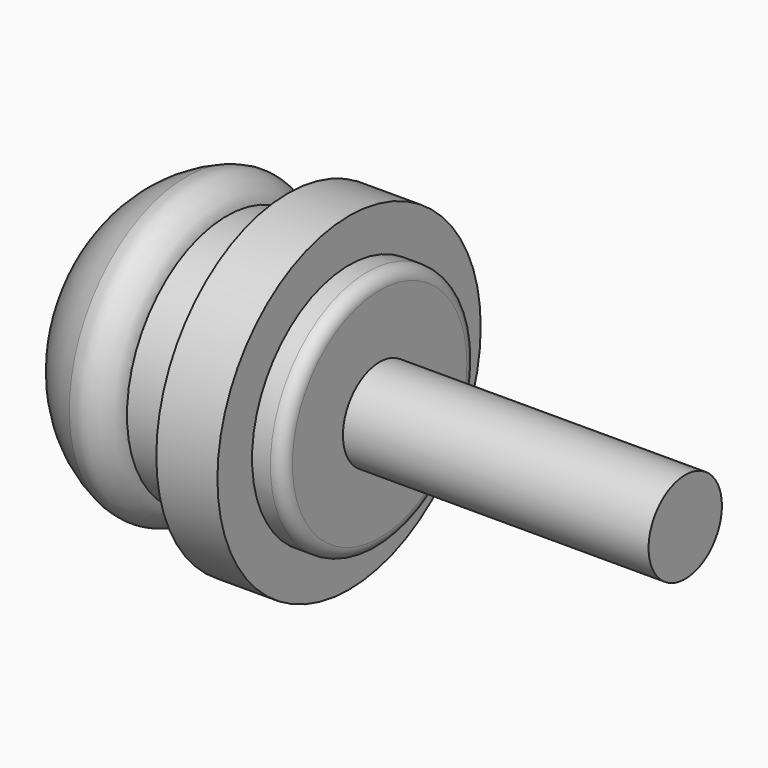
from build123d import *

# Parameters (mm, degrees)
F0_R      = 25
F1_DEPTH  = 20
F2_R      = 19.99999
F3_R      = 5
F4_R      = 20.4165647278
F5_DEPTH  = 10
F6_R      = 26.9213297652
F7_DEPTH  = 10
F8_R      = 19.8358108325
F9_DEPTH  = 5
F10_R     = 2
F11_R     = 7.5
F12_DEPTH = 50


# Not quite as in the source:
# - a fillet or chamfer is up to 0.001 mm smaller than in the source, because OpenCascade refuses the exact size


with BuildPart() as f1:
    # F0 (on Right) → F1 (new body)
    with BuildSketch(Plane.YZ):
        Circle(F0_R)
    extrude(amount=F1_DEPTH)

    # F2 (radius 20 in the source; OpenCascade refuses exactly that, so slightly less here)
    f2_edges = [f1.edges().sort_by_distance(p)[0] for p in [
        (0, -25, 0),
    ]]
    fillet(f2_edges, radius=F2_R)

    # F3
    f3_edges = [f1.edges().sort_by_distance(p)[0] for p in [
        (20, -25, 0),
    ]]
    fillet(f3_edges, radius=F3_R)

    # F4 (on face) → F5 (join)
    with BuildSketch(Plane.YZ.offset(20)):
        Circle(F4_R)
    extrude(amount=F5_DEPTH)

    # F6 (on face) → F7 (join)
    with BuildSketch(Plane.YZ.offset(30)):
        Circle(F6_R)
    extrude(amount=F7_DEPTH)

    # F8 (on face) → F9 (join)
    with BuildSketch(Plane.YZ.offset(40)):
        Circle(F8_R)
    extrude(amount=F9_DEPTH)

    # F10
    f10_edges = [f1.edges().sort_by_distance(p)[0] for p in [
        (45, -19.835811, 0),
    ]]
    fillet(f10_edges, radius=F10_R)

    # F11 (on face) → F12 (join)
    with BuildSketch(Plane.YZ.offset(45)):
        Circle(F11_R)
    extrude(amount=F12_DEPTH)


solid = f1.part
